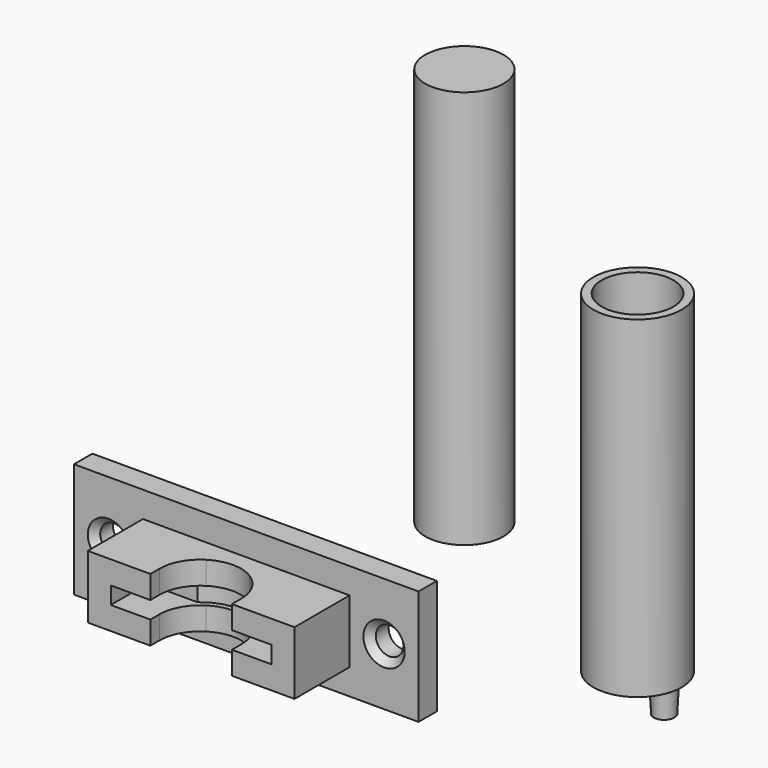
from build123d import *

# Parameters (mm, degrees)
F0_R      = 9.7663
F0_R_2    = 2.6035
F0_R_3    = 1.9304
F1_DEPTH  = 73.533
F2_R      = 7.9375
F3_DEPTH  = 73.406
F4_DEPTH  = 12.7
F4_TAPER  = 3
F5_DEPTH  = 25.4
F6_R      = 8.6614
F7_DEPTH  = 88.1634
F9_DEPTH  = 5.08
F10_DEPTH = 8.89
F11_START = 8.89
F11_DEPTH = 5.08
F12_W     = 76.2
F12_H     = 25.4
F12_R     = 3.048
F12_W_2   = 45.72
F12_H_2   = 13.97
F13_DEPTH = 5.08
F14_SIZE  = 1.524


# Not quite as in the source:
# - a feature names something its author has since deleted; it is built from what else it names


with BuildPart() as f1:
    # F0 (on Top) → F1 (new body)
    with BuildSketch(Plane.XY):
        Circle(F0_R)
        with Locations((5.8928, 0)):
            Circle(F0_R_2, mode=Mode.SUBTRACT)
        with Locations((5.8928, 0)):
            Circle(F0_R_2)
        with Locations((5.8928, 0)):
            Circle(F0_R_3, mode=Mode.SUBTRACT)
        with Locations((5.8928, 0)):
            Circle(F0_R_3)
    extrude(amount=F1_DEPTH)

    # F2 (on face) → F3 (cut)
    with BuildSketch(Plane.XY.offset(73.533)):
        Circle(F2_R)
    extrude(amount=-F3_DEPTH, mode=Mode.SUBTRACT)

    # F0 (on Top) → F4 (join)
    with BuildSketch(Plane.XY):
        with Locations((5.8928, 0)):
            Circle(F0_R_2)
        with Locations((5.8928, 0)):
            Circle(F0_R_3, mode=Mode.SUBTRACT)
    extrude(amount=-F4_DEPTH, taper=F4_TAPER)

    # F0 (on Top) → F5 (cut)
    with BuildSketch(Plane.XY):
        with Locations((5.8928, 0)):
            Circle(F0_R_3)
    extrude(amount=F5_DEPTH, mode=Mode.SUBTRACT)


with BuildPart() as f7:
    # F6 (on Top) → F7 (new body)
    with BuildSketch(Plane.XY):
        with Locations((-58.1890903413, 24.8557813466)):
            Circle(F6_R)
    extrude(amount=F7_DEPTH)


with BuildPart() as f9:
    # F8 (on Top) → F9 (new body)
    with BuildSketch(Plane.XY):
        with BuildLine():
            ThreePointArc((-69.332061944, -34.9999098742), (-62.6118536139, -32.4599098742), (-55.8916452837, -34.9999098742))
            Line((-55.8916452837, -34.9999098742), (-44.8318536139, -34.9999098742))
            Line((-44.8318536139, -34.9999098742), (-44.8318536139, -45.1599098742))
            Line((-44.8318536139, -45.1599098742), (-39.7518536139, -45.1599098742))
            Line((-39.7518536139, -45.1599098742), (-39.7518536139, -29.9199098742))
            Line((-39.7518536139, -29.9199098742), (-85.4718536139, -29.9199098742))
            Line((-85.4718536139, -29.9199098742), (-85.4718536139, -45.1599098742))
            Line((-85.4718536139, -45.1599098742), (-80.3918536139, -45.1599098742))
            Line((-80.3918536139, -45.1599098742), (-80.3918536139, -34.9999098742))
            Line((-80.3918536139, -34.9999098742), (-69.332061944, -34.9999098742))
        make_face()
        with BuildLine():
            Line((-72.7718536139, -45.1599098742), (-72.4492313132, -45.1599098742))
            ThreePointArc((-72.4492313132, -45.1599098742), (-72.6908753279, -43.9001134858), (-72.7718536139, -42.6199098742))
            Line((-72.7718536139, -42.6199098742), (-72.7718536139, -45.1599098742))
        make_face()
        with BuildLine():
            ThreePointArc((-52.4518536139, -42.6199098742), (-52.5328318998, -43.9001134858), (-52.7744759145, -45.1599098742))
            Line((-52.7744759145, -45.1599098742), (-52.4518536139, -45.1599098742))
            Line((-52.4518536139, -45.1599098742), (-52.4518536139, -42.6199098742))
        make_face()
        with BuildLine():
            ThreePointArc((-72.7718536139, -42.6199098742), (-71.872061944, -38.4397015441), (-69.332061944, -34.9999098742))
            Line((-69.332061944, -34.9999098742), (-80.3918536139, -34.9999098742))
            Line((-80.3918536139, -34.9999098742), (-80.3918536139, -45.1599098742))
            Line((-80.3918536139, -45.1599098742), (-72.7718536139, -45.1599098742))
            Line((-72.7718536139, -45.1599098742), (-72.7718536139, -42.6199098742))
        make_face()
        with BuildLine():
            Line((-44.8318536139, -34.9999098742), (-55.8916452837, -34.9999098742))
            ThreePointArc((-55.8916452837, -34.9999098742), (-53.3516452837, -38.4397015441), (-52.4518536139, -42.6199098742))
            Line((-52.4518536139, -42.6199098742), (-52.4518536139, -45.1599098742))
            Line((-52.4518536139, -45.1599098742), (-44.8318536139, -45.1599098742))
            Line((-44.8318536139, -45.1599098742), (-44.8318536139, -34.9999098742))
        make_face()
        with BuildLine():
            ThreePointArc((-67.4328378495, -34.9999098742), (-62.6118536139, -33.6029098742), (-57.7908693782, -34.9999098742))
            Line((-57.7908693782, -34.9999098742), (-55.8916452837, -34.9999098742))
            ThreePointArc((-55.8916452837, -34.9999098742), (-62.6118536139, -32.4599098742), (-69.332061944, -34.9999098742))
            Line((-69.332061944, -34.9999098742), (-67.4328378495, -34.9999098742))
        make_face()
        with BuildLine():
            Line((-71.6288536139, -45.1599098742), (-71.6288536139, -42.6199098742))
            ThreePointArc((-71.6288536139, -42.6199098742), (-70.5104960242, -38.2704573714), (-67.4328378495, -34.9999098742))
            Line((-67.4328378495, -34.9999098742), (-69.332061944, -34.9999098742))
            ThreePointArc((-69.332061944, -34.9999098742), (-71.872061944, -38.4397015441), (-72.7718536139, -42.6199098742))
            ThreePointArc((-72.7718536139, -42.6199098742), (-72.6908753279, -43.9001134858), (-72.4492313132, -45.1599098742))
            Line((-72.4492313132, -45.1599098742), (-71.6288536139, -45.1599098742))
        make_face()
        with BuildLine():
            ThreePointArc((-57.7908693782, -34.9999098742), (-54.7132112035, -38.2704573714), (-53.5948536139, -42.6199098742))
            Line((-53.5948536139, -42.6199098742), (-53.5948536139, -45.1599098742))
            Line((-53.5948536139, -45.1599098742), (-52.7744759145, -45.1599098742))
            ThreePointArc((-52.7744759145, -45.1599098742), (-52.5328318998, -43.9001134858), (-52.4518536139, -42.6199098742))
            ThreePointArc((-52.4518536139, -42.6199098742), (-53.3516452837, -38.4397015441), (-55.8916452837, -34.9999098742))
            Line((-55.8916452837, -34.9999098742), (-57.7908693782, -34.9999098742))
        make_face()
    extrude(amount=F9_DEPTH)

    # F8 (on Top) → F10 (join)
    with BuildSketch(Plane.XY):
        with BuildLine():
            ThreePointArc((-69.332061944, -34.9999098742), (-62.6118536139, -32.4599098742), (-55.8916452837, -34.9999098742))
            Line((-55.8916452837, -34.9999098742), (-44.8318536139, -34.9999098742))
            Line((-44.8318536139, -34.9999098742), (-44.8318536139, -45.1599098742))
            Line((-44.8318536139, -45.1599098742), (-39.7518536139, -45.1599098742))
            Line((-39.7518536139, -45.1599098742), (-39.7518536139, -29.9199098742))
            Line((-39.7518536139, -29.9199098742), (-85.4718536139, -29.9199098742))
            Line((-85.4718536139, -29.9199098742), (-85.4718536139, -45.1599098742))
            Line((-85.4718536139, -45.1599098742), (-80.3918536139, -45.1599098742))
            Line((-80.3918536139, -45.1599098742), (-80.3918536139, -34.9999098742))
            Line((-80.3918536139, -34.9999098742), (-69.332061944, -34.9999098742))
        make_face()
    extrude(amount=F10_DEPTH)

    # F8 (on Top) → F11 (join)
    with BuildSketch(Plane.XY.offset(F11_START)):
        with BuildLine():
            ThreePointArc((-69.332061944, -34.9999098742), (-62.6118536139, -32.4599098742), (-55.8916452837, -34.9999098742))
            Line((-55.8916452837, -34.9999098742), (-44.8318536139, -34.9999098742))
            Line((-44.8318536139, -34.9999098742), (-44.8318536139, -45.1599098742))
            Line((-44.8318536139, -45.1599098742), (-39.7518536139, -45.1599098742))
            Line((-39.7518536139, -45.1599098742), (-39.7518536139, -29.9199098742))
            Line((-39.7518536139, -29.9199098742), (-85.4718536139, -29.9199098742))
            Line((-85.4718536139, -29.9199098742), (-85.4718536139, -45.1599098742))
            Line((-85.4718536139, -45.1599098742), (-80.3918536139, -45.1599098742))
            Line((-80.3918536139, -45.1599098742), (-80.3918536139, -34.9999098742))
            Line((-80.3918536139, -34.9999098742), (-69.332061944, -34.9999098742))
        make_face()
        with BuildLine():
            Line((-44.8318536139, -34.9999098742), (-55.8916452837, -34.9999098742))
            ThreePointArc((-55.8916452837, -34.9999098742), (-53.3516452837, -38.4397015441), (-52.4518536139, -42.6199098742))
            Line((-52.4518536139, -42.6199098742), (-52.4518536139, -45.1599098742))
            Line((-52.4518536139, -45.1599098742), (-44.8318536139, -45.1599098742))
            Line((-44.8318536139, -45.1599098742), (-44.8318536139, -34.9999098742))
        make_face()
        with BuildLine():
            ThreePointArc((-67.4328378495, -34.9999098742), (-62.6118536139, -33.6029098742), (-57.7908693782, -34.9999098742))
            Line((-57.7908693782, -34.9999098742), (-55.8916452837, -34.9999098742))
            ThreePointArc((-55.8916452837, -34.9999098742), (-62.6118536139, -32.4599098742), (-69.332061944, -34.9999098742))
            Line((-69.332061944, -34.9999098742), (-67.4328378495, -34.9999098742))
        make_face()
        with BuildLine():
            ThreePointArc((-72.7718536139, -42.6199098742), (-71.872061944, -38.4397015441), (-69.332061944, -34.9999098742))
            Line((-69.332061944, -34.9999098742), (-80.3918536139, -34.9999098742))
            Line((-80.3918536139, -34.9999098742), (-80.3918536139, -45.1599098742))
            Line((-80.3918536139, -45.1599098742), (-72.7718536139, -45.1599098742))
            Line((-72.7718536139, -45.1599098742), (-72.7718536139, -42.6199098742))
        make_face()
        with BuildLine():
            Line((-72.7718536139, -45.1599098742), (-72.4492313132, -45.1599098742))
            ThreePointArc((-72.4492313132, -45.1599098742), (-72.6908753279, -43.9001134858), (-72.7718536139, -42.6199098742))
            Line((-72.7718536139, -42.6199098742), (-72.7718536139, -45.1599098742))
        make_face()
        with BuildLine():
            ThreePointArc((-52.4518536139, -42.6199098742), (-52.5328318998, -43.9001134858), (-52.7744759145, -45.1599098742))
            Line((-52.7744759145, -45.1599098742), (-52.4518536139, -45.1599098742))
            Line((-52.4518536139, -45.1599098742), (-52.4518536139, -42.6199098742))
        make_face()
        with BuildLine():
            Line((-71.6288536139, -45.1599098742), (-71.6288536139, -42.6199098742))
            ThreePointArc((-71.6288536139, -42.6199098742), (-70.5104960242, -38.2704573714), (-67.4328378495, -34.9999098742))
            Line((-67.4328378495, -34.9999098742), (-69.332061944, -34.9999098742))
            ThreePointArc((-69.332061944, -34.9999098742), (-71.872061944, -38.4397015441), (-72.7718536139, -42.6199098742))
            ThreePointArc((-72.7718536139, -42.6199098742), (-72.6908753279, -43.9001134858), (-72.4492313132, -45.1599098742))
            Line((-72.4492313132, -45.1599098742), (-71.6288536139, -45.1599098742))
        make_face()
        with BuildLine():
            ThreePointArc((-57.7908693782, -34.9999098742), (-54.7132112035, -38.2704573714), (-53.5948536139, -42.6199098742))
            Line((-53.5948536139, -42.6199098742), (-53.5948536139, -45.1599098742))
            Line((-53.5948536139, -45.1599098742), (-52.7744759145, -45.1599098742))
            ThreePointArc((-52.7744759145, -45.1599098742), (-52.5328318998, -43.9001134858), (-52.4518536139, -42.6199098742))
            ThreePointArc((-52.4518536139, -42.6199098742), (-53.3516452837, -38.4397015441), (-55.8916452837, -34.9999098742))
            Line((-55.8916452837, -34.9999098742), (-57.7908693782, -34.9999098742))
        make_face()
    extrude(amount=F11_DEPTH)

    # F12 (on face) → F13 (join)
    with BuildSketch(Plane(origin=(0, -29.9199098742, 0), x_dir=(-1, 0, 0), z_dir=(0, 1, 0))):
        with Locations((62.6118536139, 6.985)):
            Rectangle(F12_W, F12_H)
        with Locations((32.1318536139, 6.985)):
            Circle(F12_R, mode=Mode.SUBTRACT)
        with Locations((62.6118536139, 6.985)):
            Rectangle(F12_W_2, F12_H_2, mode=Mode.SUBTRACT)
        with Locations((93.0918536139, 6.985)):
            Circle(F12_R, mode=Mode.SUBTRACT)
        with Locations((62.6118536139, 6.985)):
            Rectangle(F12_W_2, F12_H_2)
    extrude(amount=F13_DEPTH)

    # F14
    f14_edges = [f9.edges().sort_by_distance(p)[0] for p in [
        (-90.043854, -29.91991, 6.985),
        (-29.083854, -29.91991, 6.985),
    ]]
    chamfer(f14_edges, length=F14_SIZE)


solid = Compound([f1.part, f7.part, f9.part])
